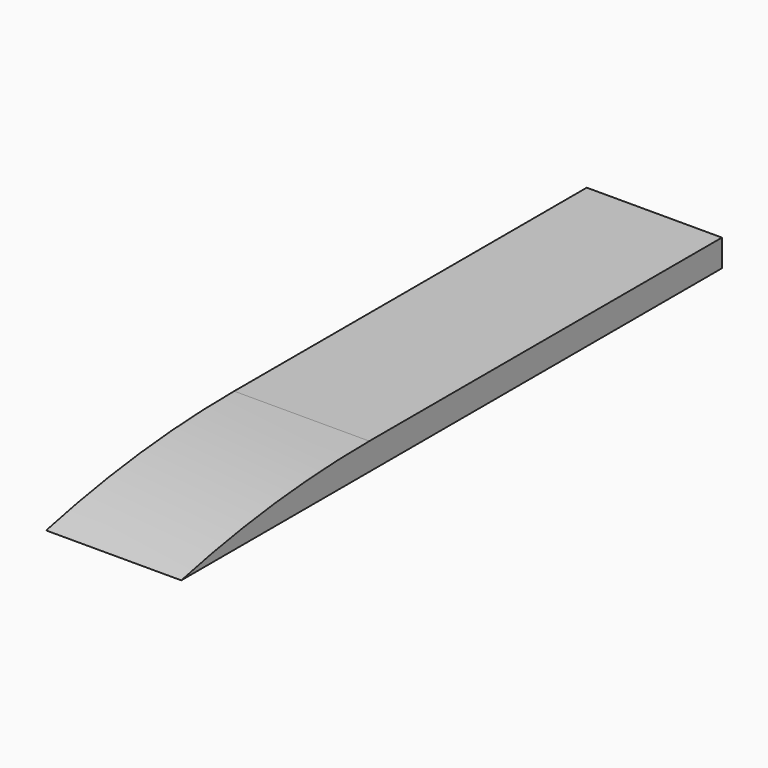
from build123d import *

# Parameters (mm, degrees)
F0_W        = 38.1
F0_H        = 190.5
F1_DEPTH    = 7.62
F2_T1_DEPTH = 369.3970678465


# Not quite as in the source:
# - a fillet or chamfer that OpenCascade refuses, or shapes differently, is made with other operations: its cross-section is extruded or revolved along the edge and cut away or added


with BuildPart() as f1:
    # F0 (on Top) → F1 (new body)
    with BuildSketch(Plane.XY):
        with Locations((-7.4515999526, -95.25)):
            Rectangle(F0_W, F0_H)
    extrude(amount=F1_DEPTH)

    # F2: fillet of radius 291.8880765452 on 1 edges, made by hand

    # F2_s2 → F2_t1 (cut)
    with BuildSketch(Plane.YZ.offset(-192.1501338759)):
        with BuildLine():
            ThreePointArc((-190.5, 0), (-157.5886534157, 5.7087426277), (-124.2405864307, 7.62))
            Line((-124.2405864307, 7.62), (-124.2405864307, 13.4577615309))
            Line((-124.2405864307, 13.4577615309), (-190.5, 13.4577615309))
            Line((-190.5, 13.4577615309), (-196.3377615309, 7.62))
            ThreePointArc((-196.3377615309, 7.62), (-196.3377615309, 3.81), (-191.8251882714, 5.6853615309))
            Line((-191.8251882714, 5.6853615309), (-190.5, 0))
        make_face()
    extrude(amount=F2_T1_DEPTH, mode=Mode.SUBTRACT)


solid = f1.part
